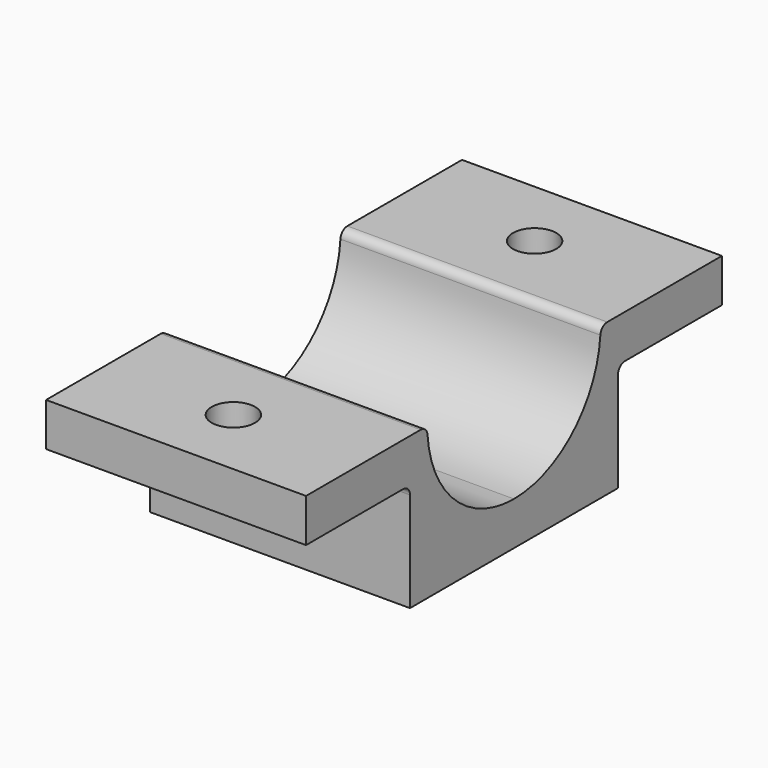
from build123d import *

# Parameters (mm, degrees)
F0_W     = 30
F0_H     = 30
F1_DEPTH = 5
F2_W     = 15
F2_H     = 5
F3_DEPTH = 30
F4_R     = 1
F6_D     = 5


with BuildPart() as f1:
    # F0 (on Top) → F1 (new body)
    with BuildSketch(Plane.XY):
        Rectangle(F0_W, F0_H)
    extrude(amount=-F1_DEPTH)

    # F2 (on face) → F3 (join)
    with BuildSketch(Plane(origin=(-15, 0, 0), x_dir=(0, -1, 0), z_dir=(-1, 0, 0))):
        with Locations((-22.5, 10)):
            Rectangle(F2_W, F2_H)
        with BuildLine():
            ThreePointArc((0, 0), (-8.8388347648, 3.6611652352), (-12.5, 12.5))
            Line((-12.5, 12.5), (-15, 12.5))
            Line((-15, 12.5), (-15, 7.5))
            Line((-15, 7.5), (-15, 0))
            Line((-15, 0), (0, 0))
        make_face()
        with BuildLine():
            ThreePointArc((12.5, 12.5), (8.8388347648, 3.6611652352), (0, 0))
            Line((0, 0), (15, 0))
            Line((15, 0), (15, 7.5))
            Line((15, 7.5), (15, 12.5))
            Line((15, 12.5), (12.5, 12.5))
        make_face()
        with Locations((22.5, 10)):
            Rectangle(F2_W, F2_H)
    extrude(amount=-F3_DEPTH)

    # F4
    f4_edges = [f1.edges().sort_by_distance(p)[0] for p in [
        (0, 12.5, 12.5),
        (0, -15, 7.5),
        (0, 15, 7.5),
        (0, -12.5, 12.5),
    ]]
    fillet(f4_edges, radius=F4_R)

    # F6 (through all)
    with Locations(Plane.XY.offset(12.5)):
        with Locations((0, 21.7314560089), (0, -21.7314560089)):
            Hole(F6_D / 2)


solid = f1.part
